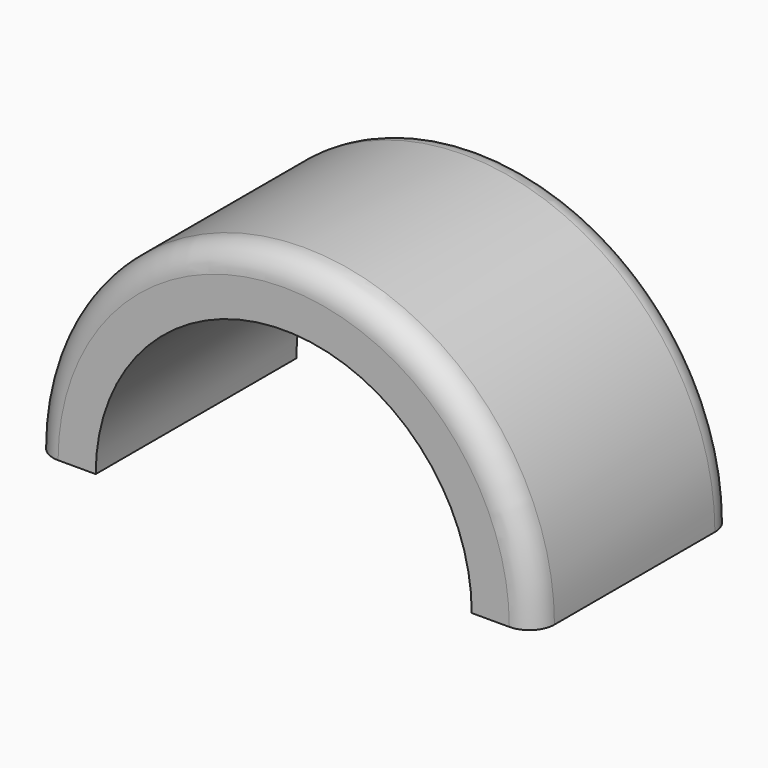
from build123d import *

# Parameters (mm, degrees)
F1_DEPTH = 10
F2_R     = 1
F3_R     = 0.6
F4_DEPTH = 2.5


with BuildPart() as f1:
    # F0 (on Front) → F1 (new body)
    with BuildSketch(Plane.XZ):
        with BuildLine():
            Line((7.5, 55.5), (10, 55.5))
            ThreePointArc((10, 55.5), (0, 65.5), (-10, 55.5))
            Line((-10, 55.5), (-7.5, 55.5))
            ThreePointArc((-7.5, 55.5), (0, 63), (7.5, 55.5))
        make_face()
    extrude(amount=F1_DEPTH)

    # F2
    f2_edges = [f1.edges().sort_by_distance(p)[0] for p in [
        (0, 0, 65.5),
        (0, -10, 65.5),
    ]]
    fillet(f2_edges, radius=F2_R)

    # F3 (on face) → F4 (cut)
    with BuildSketch(Plane(origin=(0, 0, 55.5), x_dir=(1, 0, 0), z_dir=(0, 0, -1))):
        with Locations((8.75, 1.5)):
            Circle(F3_R)
        with Locations((8.75, 8.5)):
            Circle(F3_R)
        with Locations((-8.75, 1.5)):
            Circle(F3_R)
        with Locations((-8.75, 8.5)):
            Circle(F3_R)
    extrude(amount=-F4_DEPTH, mode=Mode.SUBTRACT)


solid = f1.part
